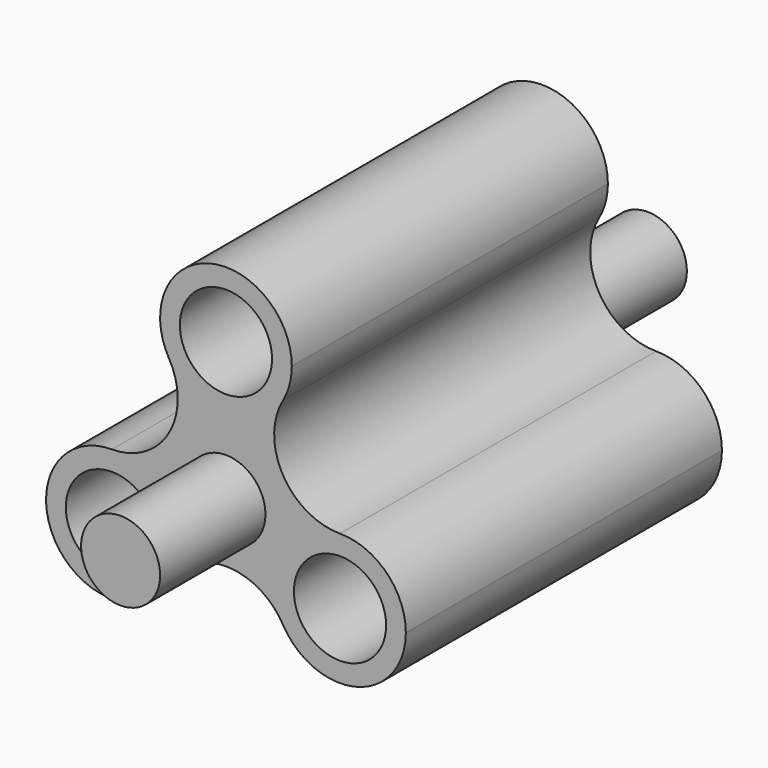
from build123d import *

# Parameters (mm, degrees)
F0_R          = 3.5
F1_DEPTH      = 30
F2_R          = 3
F3_DEPTH      = 40
F3_DEPTH_BACK = 10


# Not quite as in the source:
# - ends of sketch curves that miss each other by under 0.0002 mm in the source are joined


with BuildPart() as f1:
    # F0 (on Front) → F1 (new body)
    with BuildSketch(Plane.XZ):
        with BuildLine():
            ThreePointArc((-4.3301281481, 8.0578746702), (-6.557e-07, 5.5578757428), (4.330125744, 8.057876563))
            ThreePointArc((4.330125744, 8.057876563), (4.8296291409, 9.2637805524), (5, 10.5578757428))
            ThreePointArc((5, 10.5578757428), (-1.2940954014, 15.3875048271), (-4.3301281481, 8.0578746702))
        make_face()
        with Locations((0, 10.5578757428)):
            Circle(F0_R, mode=Mode.SUBTRACT)
        with BuildLine():
            ThreePointArc((8.6602543293, 0.557875869), (4.3301271646, 3.0578757428), (4.3301270553, 8.0578758059))
            ThreePointArc((4.3301270553, 8.0578758059), (-6.557e-07, 5.5578757428), (-4.3301281481, 8.0578746702))
            ThreePointArc((-4.3301281481, 8.0578746702), (-4.330127711, 3.0578747964), (-8.6602543293, 0.5578743547))
            ThreePointArc((-8.6602543293, 0.5578743547), (-5.1247199995, -0.9065915075), (-3.6602536736, -4.4421256453))
            ThreePointArc((-3.6602536736, -4.4421256453), (-3.8306244761, -5.7362206245), (-4.3301263997, -6.9421252036))
            ThreePointArc((-4.3301263997, -6.9421252036), (4.371e-07, -4.442124762), (4.330127711, -6.9421244465))
            ThreePointArc((4.330127711, -6.9421244465), (4.3301273832, -1.9421243834), (8.6602543293, 0.557875869))
        make_face()
        with BuildLine():
            ThreePointArc((13.6602545478, -4.442124131), (12.1957883765, -0.9065901478), (8.6602543293, 0.557875869))
            ThreePointArc((8.6602543293, 0.557875869), (4.3301273832, -1.9421243834), (4.330127711, -6.9421244465))
            ThreePointArc((4.330127711, -6.9421244465), (9.9543499492, -9.2717532153), (13.6602545478, -4.442124131))
        make_face()
        with Locations((8.6602545478, -4.442124131)):
            Circle(F0_R, mode=Mode.SUBTRACT)
        with BuildLine():
            ThreePointArc((-3.6602536736, -4.4421256453), (-5.1247199995, -0.9065915075), (-8.6602543293, 0.5578743547))
            ThreePointArc((-8.6602543293, 0.5578743547), (-12.9903804011, -6.94212615), (-4.3301263997, -6.9421252036))
            ThreePointArc((-4.3301263997, -6.9421252036), (-3.8306244761, -5.7362206245), (-3.6602536736, -4.4421256453))
        make_face()
        with Locations((-8.6602536736, -4.4421256453)):
            Circle(F0_R, mode=Mode.SUBTRACT)
    extrude(amount=F1_DEPTH)

    # F2 (on Front) → F3 (join, two sides)
    with BuildSketch(Plane.XZ) as f3_sk:
        Circle(F2_R)
    extrude(amount=F3_DEPTH)
    extrude(f3_sk.sketch, amount=-F3_DEPTH_BACK)


solid = f1.part
